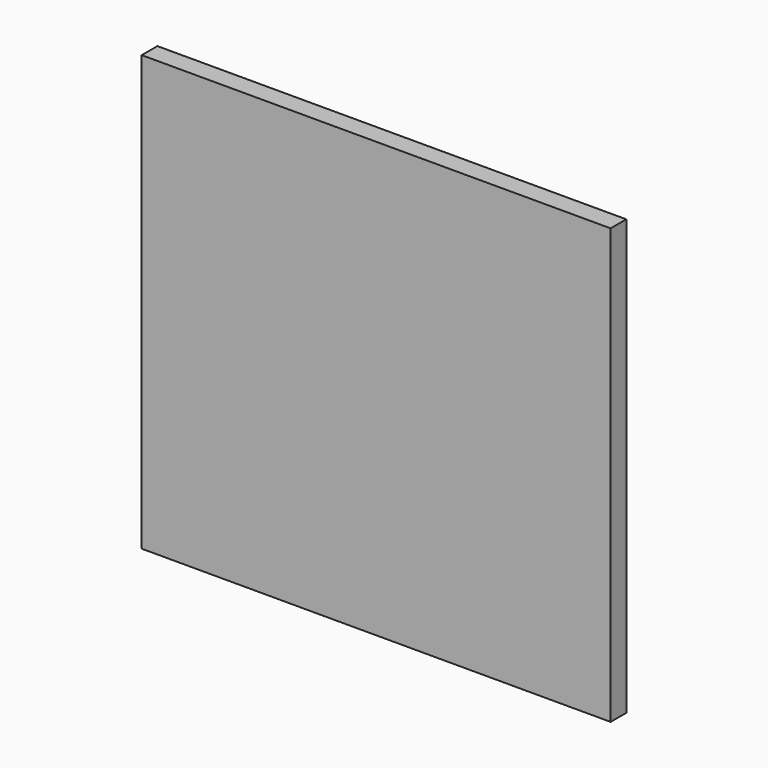
from build123d import *

# Parameters (mm, degrees)
F0_W     = 455.676
F0_H     = 396.875
F1_DEPTH = 19.05
F2_DEPTH = 25.4


# Not quite as in the source:
# - a feature names something its author has since deleted; it is built from what else it names


with BuildPart() as f1:
    # F0 (on Front) → F1 (new body)
    with BuildSketch(Plane.XZ):
        with Locations((-229.362, 0)):
            Rectangle(F0_W, F0_H)
    extrude(amount=F1_DEPTH)

    # F2 (add): a face of the model
    f2_faces = [f1.faces().sort_by_distance(p)[0] for p in [
        (-229.362, -9.525, 198.4375),
    ]]
    extrude(f2_faces, amount=F2_DEPTH)


solid = f1.part
